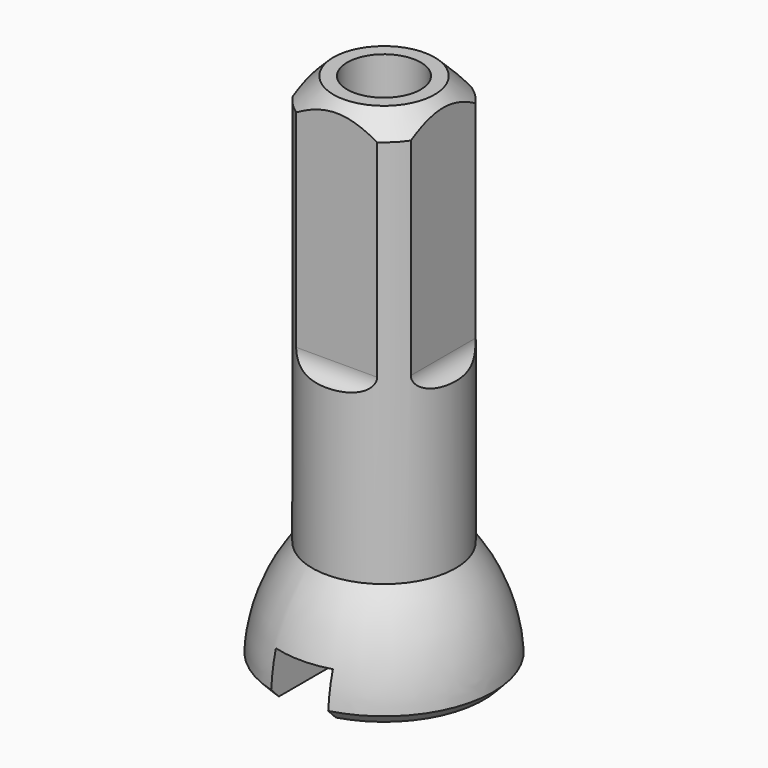
from build123d import *

# Parameters (mm, degrees)
F2_R         = 7.5
F2_W         = 3.22
F2_H         = 3.22
F3_DEPTH     = 6.7
F4_T4_DEPTH  = 4.7003636063
F4_S5_R      = 1.95
F4_T6_DEPTH  = 4
F4_T10_DEPTH = 4.7003636063
F4_S11_R     = 1.95
F4_T12_DEPTH = 4
F4_T16_DEPTH = 4.7003636063
F4_S17_R     = 1.95
F4_T18_DEPTH = 4
F4_T22_DEPTH = 4.7003636063
F4_S23_R     = 1.95
F4_T24_DEPTH = 4
F6_R         = 1
F7_DEPTH     = 14.051
F10_W        = 1.55
F10_H        = 10
F11_DEPTH    = 1.2


# Not quite as in the source:
# - a fillet or chamfer that OpenCascade refuses, or shapes differently, is made with other operations: its cross-section is extruded or revolved along the edge and cut away or added


with BuildPart() as f1:
    # F0 (on Right) → F1 (revolve)
    with BuildSketch(Plane.YZ):
        with BuildLine():
            Line((0, 14.05), (0, 0))
            Line((0, 0), (2.975, 0))
            ThreePointArc((2.975, 0), (2.7112109327, 1.5379064503), (1.95, 2.9))
            Line((1.95, 2.9), (1.95, 14.05))
            Line((1.95, 14.05), (0, 14.05))
        make_face()
    revolve(axis=Axis((0, 0, 7.7619114891), (0, 0, 1)))

    # F2 (on face) → F3 (cut)
    with BuildSketch(Plane.XY.offset(14.05)):
        Circle(F2_R)
        Rectangle(F2_W, F2_H, mode=Mode.SUBTRACT)
    extrude(amount=-F3_DEPTH, mode=Mode.SUBTRACT)

    # F4: fillet of radius 0.5 on 4 edges, made by hand


with BuildPart() as f4_tool2:
    # F4_s3 → F4_t4 (new body)
    with BuildSketch(Plane.XZ.offset(-2.3501818032)):
        with BuildLine():
            ThreePointArc((1.61, 7.85), (1.7564466094, 7.4964466094), (2.11, 7.35))
            Line((2.11, 7.35), (1.61, 7.35))
            Line((1.61, 7.35), (1.61, 7.85))
        make_face()
    extrude(amount=F4_T4_DEPTH)

    # F4_s5 → F4_t6 (intersect, symmetric)
    with BuildSketch(Plane.XY.offset(7.6)):
        Circle(F4_S5_R)
    extrude(amount=F4_T6_DEPTH, both=True, mode=Mode.INTERSECT)


with BuildPart() as f1_1:
    add(f1.part)

    # F4_t1: union F4_tool2
    add(f4_tool2.part)


with BuildPart() as f4_tool8:
    # F4_s9 → F4_t10 (new body)
    with BuildSketch(Plane.YZ.offset(2.3501818032)):
        with BuildLine():
            ThreePointArc((-1.61, 7.85), (-1.7564466094, 7.4964466094), (-2.11, 7.35))
            Line((-2.11, 7.35), (-1.61, 7.35))
            Line((-1.61, 7.35), (-1.61, 7.85))
        make_face()
    extrude(amount=-F4_T10_DEPTH)

    # F4_s11 → F4_t12 (intersect, symmetric)
    with BuildSketch(Plane.XY.offset(7.6)):
        Circle(F4_S11_R)
    extrude(amount=F4_T12_DEPTH, both=True, mode=Mode.INTERSECT)


with BuildPart() as f1_2:
    add(f1_1.part)

    # F4_t7: union F4_tool8
    add(f4_tool8.part)


with BuildPart() as f4_tool14:
    # F4_s15 → F4_t16 (new body)
    with BuildSketch(Plane.YZ.offset(-2.3501818032)):
        with BuildLine():
            ThreePointArc((2.11, 7.35), (1.7564466094, 7.4964466094), (1.61, 7.85))
            Line((1.61, 7.85), (1.61, 7.35))
            Line((1.61, 7.35), (2.11, 7.35))
        make_face()
    extrude(amount=F4_T16_DEPTH)

    # F4_s17 → F4_t18 (intersect, symmetric)
    with BuildSketch(Plane.XY.offset(7.6)):
        Circle(F4_S17_R)
    extrude(amount=F4_T18_DEPTH, both=True, mode=Mode.INTERSECT)


with BuildPart() as f1_3:
    add(f1_2.part)

    # F4_t13: union F4_tool14
    add(f4_tool14.part)


with BuildPart() as f4_tool20:
    # F4_s21 → F4_t22 (new body)
    with BuildSketch(Plane.XZ.offset(2.3501818032)):
        with BuildLine():
            ThreePointArc((-1.61, 7.85), (-1.7564466094, 7.4964466094), (-2.11, 7.35))
            Line((-2.11, 7.35), (-1.61, 7.35))
            Line((-1.61, 7.35), (-1.61, 7.85))
        make_face()
    extrude(amount=-F4_T22_DEPTH)

    # F4_s23 → F4_t24 (intersect, symmetric)
    with BuildSketch(Plane.XY.offset(7.6)):
        Circle(F4_S23_R)
    extrude(amount=F4_T24_DEPTH, both=True, mode=Mode.INTERSECT)


with BuildPart() as f1_4:
    add(f1_3.part)

    # F4_t19: union F4_tool20
    add(f4_tool20.part)

    # F5: chamfer of 0.25 on 1 edges, made by hand

    # F5_s1 → F5_t2 (revolve, cut)
    with BuildSketch(Plane.YZ):
        with BuildLine():
            Line((2.9674244141, 0.2643186422), (2.7178347979, 0))
            Line((2.7178347979, 0), (2.975, 0))
            ThreePointArc((2.975, 0), (2.9730031083, 0.135746377), (2.9674244141, 0.2643186422))
        make_face()
    revolve(axis=Axis((0, 0, 0), (0, 0, 1)), mode=Mode.SUBTRACT)

    # F6 (on face) → F7 (cut, through all)
    with BuildSketch(Plane.XY.offset(14.05)):
        Circle(F6_R)
    extrude(amount=-F7_DEPTH, mode=Mode.SUBTRACT)

    # F8 (on Front) → F9 (revolve, cut)
    with BuildSketch(Plane.XZ):
        Polygon((-3.375, 12.05), (-1.375, 14.05), (-3.375, 14.05), align=None)
    revolve(axis=Axis((0, 0, 9.9016753957), (0, 0, 1)), mode=Mode.SUBTRACT)

    # F10 (on face) → F11 (cut)
    with BuildSketch(Plane(origin=(0, 0, 0), x_dir=(1, 0, 0), z_dir=(0, 0, -1))):
        Rectangle(F10_W, F10_H)
    extrude(amount=-F11_DEPTH, mode=Mode.SUBTRACT)


solid = f1_4.part
